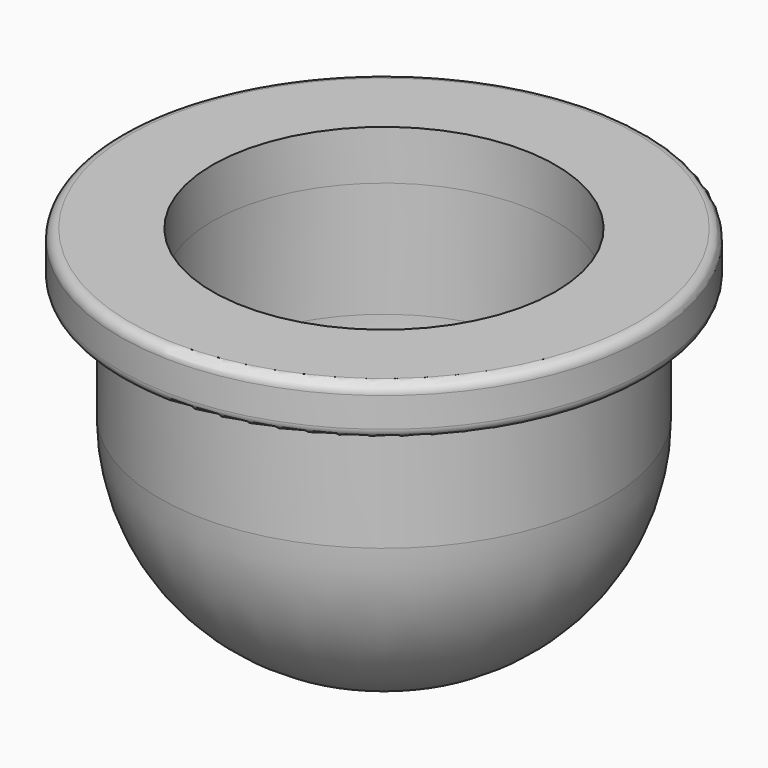
from build123d import *

# Parameters (mm, degrees)
F2_R = 6.3
F3_R = 0.3
F4_T = 1.6


# Not quite as in the source:
# - a shell that OpenCascade refuses in one call is made with other operations: the cavity is built on its own and cut out


with BuildPart() as f1:
    # F0 (on Front) → F1 (revolve)
    with BuildSketch(Plane.XZ):
        Polygon((8, 0), (0, 0), (0, -11.3), (6.8, -11.3), (6.8, -1.5), (8, -1.5), align=None)
    revolve(axis=Axis((0, 0, -5.65), (0, 0, -1)))

    # F2
    f2_edges = [f1.edges().sort_by_distance(p)[0] for p in [
        (-6.8, 0, -11.3),
    ]]
    fillet(f2_edges, radius=F2_R)

    # F3
    f3_edges = [f1.edges().sort_by_distance(p)[0] for p in [
        (-8, 0, -1.5),
        (-8, 0, 0),
        (8, 0, -0.75),
    ]]
    fillet(f3_edges, radius=F3_R)

    # F4: shell of thickness 1.6, made by hand


with BuildPart() as f4_core1:
    # F4_t2: copy of F1
    add(f1.part)

    # the walls: a layer under each face that stays
    f4_faces = [f4_core1.faces().sort_by_distance(p)[0] for p in [
        (5.1333333333, 5.1333333333, -1.5),
        (-6.8, 0, -3.25),
        (-8, 0, -0.75),
        (-4.9547727215, 0, -9.4547727215),
        (0, 0, -11.3),
    ]]
    thicken(f4_faces, amount=-F4_T, mode=Mode.SUBTRACT)

    # F4_s3 → F4_t4 (revolve, cut)
    with BuildSketch(Plane.XZ):
        Polygon((6.816, -1.516), (6.8, 0.1), (5.2, 0.1), (5.2, -1.5), align=None)
    revolve(axis=Axis((0, 0, -1.5), (0, 0, -1)), mode=Mode.SUBTRACT)


with BuildPart() as f1_1:
    add(f1.part)

    # what is left inside the walls is the cavity
    f4_cavity = [f4_core1.part.solids().sort_by_distance(p)[0] for p in [
        (-2.842, 0, -9.056463),
    ]]
    add(f4_cavity, mode=Mode.SUBTRACT)


solid = f1_1.part
